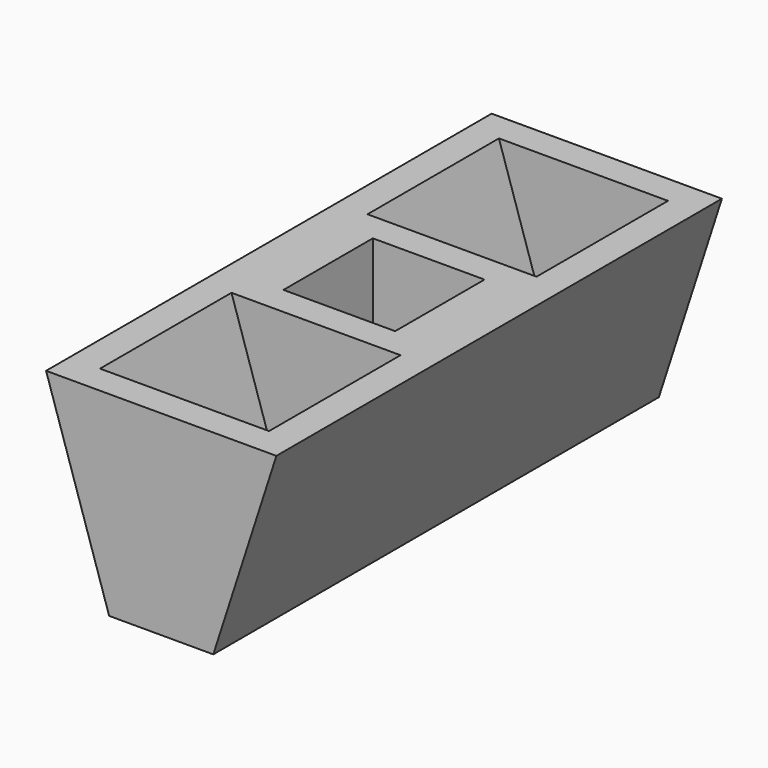
from build123d import *

# Parameters (mm, degrees)
F1_W        = 36.2
F1_H        = 68.8
F2_W        = 12.866667
F2_H        = 68.8
F4_DEPTH    = 12
F5_W        = 13.8
F5_H        = 13.8
F6_DEPTH    = 32
F7_T        = 3.6
F7_T3_DEPTH = 27.2
F7_T5_DEPTH = 21
F7_T7_DEPTH = 21


# Not quite as in the source:
# - a shell that OpenCascade refuses in one call is made with other operations: the cavity is built on its own and cut out


with BuildPart() as f3:
    # F1 (on offset) → F3 section 0
    with BuildSketch(Plane.XY.offset(36.125)):
        with Locations((0, -34.4)):
            Rectangle(F1_W, F1_H)
    # F2 (on Top) → F3 section 1
    with BuildSketch(Plane.XY):
        with Locations((-3.35e-05, -34.4)):
            Rectangle(F2_W, F2_H)
    loft()

    # F4 (cut): a face of the model
    f4_faces = [f3.faces().sort_by_distance(p)[0] for p in [
        (0, -34.4, 36.125),
    ]]
    extrude(f4_faces, amount=-F4_DEPTH, mode=Mode.SUBTRACT)

    # F5 (on offset) → F6 (cut)
    with BuildSketch(Plane.XY.offset(36.125)):
        with Locations((0, -34.4)):
            Rectangle(F5_W, F5_H)
    extrude(amount=-F6_DEPTH, mode=Mode.SUBTRACT)

    # F7: shell of thickness 3.6, made by hand


with BuildPart() as f7_core1:
    # F7_t2: copy of F3
    add(f3.part)

    # the walls: a layer under each face that stays
    f7_faces = [f7_core1.faces().sort_by_distance(p)[0] for p in [
        (-2.2314e-05, 0, 12.0625),
        (10.3289282007, -34.4, 12.0625),
        (-3.35e-05, -34.4, 0),
        (-10.3289728287, -34.4, 12.0625),
        (-2.2314e-05, -68.8, 12.0625),
        (0, -27.5, 14.125),
        (6.9, -34.4, 14.125),
        (0, -41.3, 14.125),
        (-6.9, -34.4, 14.125),
        (0, -34.4, 4.125),
    ]]
    thicken(f7_faces, amount=-F7_T, mode=Mode.SUBTRACT)

    # F7_s4 → F7_t3 (cut)
    with BuildSketch(Plane.XY.offset(0.525)):
        Polygon((-6.864, -27.536), (-6.9, -23.9), (-10.5, -23.9), (-10.5, -27.5), align=None)
        Polygon((6.864, -27.536), (6.9, -23.9), (10.5, -23.9), (10.5, -27.5), align=None)
        Polygon((6.864, -41.264), (10.5, -41.3), (10.5, -44.9), (6.9, -44.9), align=None)
        Polygon((-6.864, -41.264), (-6.9, -44.9), (-10.5, -44.9), (-10.5, -41.3), align=None)
    extrude(amount=F7_T3_DEPTH, mode=Mode.SUBTRACT)

    # F7_s6 → F7_t5 (cut)
    with BuildSketch(Plane.YZ.offset(-10.5)):
        Polygon((-27.536, 4.161), (-23.9, 4.125), (-23.9, 0.525), (-27.5, 0.525), align=None)
        Polygon((-41.264, 4.161), (-44.9, 4.125), (-44.9, 0.525), (-41.3, 0.525), align=None)
    extrude(amount=F7_T5_DEPTH, mode=Mode.SUBTRACT)

    # F7_s8 → F7_t7 (cut)
    with BuildSketch(Plane.XZ.offset(23.9)):
        Polygon((6.864, 4.161), (10.5, 4.125), (10.5, 0.525), (6.9, 0.525), align=None)
        Polygon((-6.864, 4.161), (-10.5, 4.125), (-10.5, 0.525), (-6.9, 0.525), align=None)
    extrude(amount=F7_T7_DEPTH, mode=Mode.SUBTRACT)


with BuildPart() as f3_1:
    add(f3.part)

    # what is left inside the walls is the cavity
    f7_cavity = [f7_core1.part.solids().sort_by_distance(p)[0] for p in [
        (8.197675, -13.75, 17.294397),
        (8.197675, -55.05, 17.294397),
    ]]
    add(f7_cavity, mode=Mode.SUBTRACT)


solid = f3_1.part
